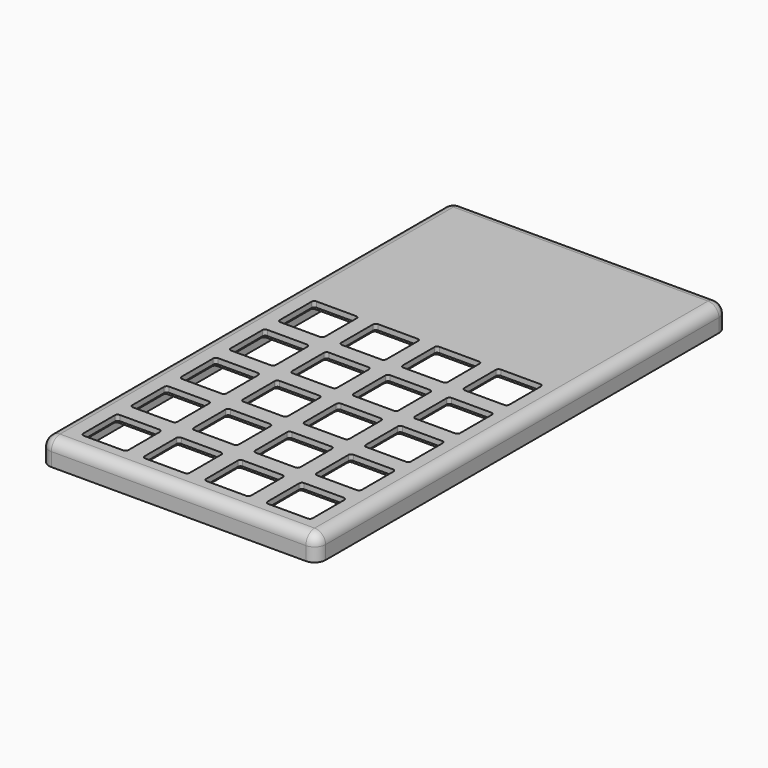
from build123d import *

# Parameters (mm, degrees)
F0_W         = 80.3275
F0_H         = 149.225
F1_DEPTH     = 7.14375
F2_R         = 3.175
F3_T1_DEPTH  = 11.90625
F3_S5_W      = 3.175
F3_S5_H      = 3.175
F3_T6_DEPTH  = 3.175
F3_S11_W     = 3.175
F3_S11_H     = 3.175
F3_T12_DEPTH = 3.175
F3_S17_W     = 3.175
F3_S17_H     = 3.175
F3_T18_DEPTH = 3.175
F3_S23_W     = 3.175
F3_S23_H     = 3.175
F3_T24_DEPTH = 3.175
F4_W         = 71.59625
F4_H         = 142.875
F5_DEPTH     = 5.55625
F7_DEPTH     = 25.4
F1_FACE_W    = 71.59625
F1_FACE_H    = 142.875
F9_DEPTH     = 25.4
F11_DEPTH    = 1.5875
F12_W        = 6.35
F12_H        = 1.984375
F12_W_2      = 12.7
F12_H_2      = 1.5875
F13_DEPTH    = 6.35


# Not quite as in the source:
# - a fillet or chamfer that OpenCascade refuses, or shapes differently, is made with other operations: its cross-section is extruded or revolved along the edge and cut away or added


with BuildPart() as f1:
    # F0 (on Top) → F1 (new body)
    with BuildSketch(Plane.XY):
        Rectangle(F0_W, F0_H)
    extrude(amount=F1_DEPTH)

    # F2
    f2_edges = [f1.edges().sort_by_distance(p)[0] for p in [
        (-40.16375, 0, 7.14375),
        (0, 74.6125, 7.14375),
        (40.16375, 0, 7.14375),
        (0, -74.6125, 7.14375),
    ]]
    fillet(f2_edges, radius=F2_R)

    # F3: fillet of radius 3.175 on 4 edges, made by hand

    # F3_s2 → F3_t1 (cut)
    with BuildSketch(Plane.XY.offset(-7.9375)):
        with BuildLine():
            ThreePointArc((40.16375, 71.4375), (39.2338140303, 73.6825640303), (36.98875, 74.6125))
            Line((36.98875, 74.6125), (40.16375, 74.6125))
            Line((40.16375, 74.6125), (40.16375, 71.4375))
        make_face()
        with BuildLine():
            ThreePointArc((40.16375, -71.4375), (39.2338140303, -73.6825640303), (36.98875, -74.6125))
            Line((36.98875, -74.6125), (40.16375, -74.6125))
            Line((40.16375, -74.6125), (40.16375, -71.4375))
        make_face()
        with BuildLine():
            ThreePointArc((-36.98875, -74.6125), (-39.2338140303, -73.6825640303), (-40.16375, -71.4375))
            Line((-40.16375, -71.4375), (-40.16375, -74.6125))
            Line((-40.16375, -74.6125), (-36.98875, -74.6125))
        make_face()
        with BuildLine():
            ThreePointArc((-36.98875, 74.6125), (-39.2338140303, 73.6825640303), (-40.16375, 71.4375))
            Line((-40.16375, 71.4375), (-40.16375, 74.6125))
            Line((-40.16375, 74.6125), (-36.98875, 74.6125))
        make_face()
    extrude(amount=F3_T1_DEPTH, mode=Mode.SUBTRACT)


with BuildPart() as f3_tool4:
    # F3_s5 → F3_t6 (new body)
    with BuildSketch(Plane.XZ.offset(-71.4375)):
        with Locations((-38.57625, 5.55625)):
            Rectangle(F3_S5_W, F3_S5_H)
    extrude(amount=-F3_T6_DEPTH)

    # F3_s7 → F3_t8 (revolve, cut)
    with BuildSketch(Plane(origin=(-36.98875, 71.4375, 3.96875), x_dir=(0.7071067812, 0, -0.7071067812), z_dir=(0.7071067812, 0, 0.7071067812))):
        with BuildLine():
            ThreePointArc((0, -3.175), (3.175, 0), (0, 3.175))
            Line((0, 3.175), (0, -3.175))
        make_face()
    revolve(axis=Axis((-36.98875, 71.4375, 3.96875), (0, 1, 0)), mode=Mode.SUBTRACT)


with BuildPart() as f1_1:
    add(f1.part)

    # F3_t3: cut F3_tool4
    add(f3_tool4.part, mode=Mode.SUBTRACT)


with BuildPart() as f3_tool10:
    # F3_s11 → F3_t12 (new body)
    with BuildSketch(Plane.XZ.offset(71.4375)):
        with Locations((-38.57625, 5.55625)):
            Rectangle(F3_S11_W, F3_S11_H)
    extrude(amount=F3_T12_DEPTH)

    # F3_s13 → F3_t14 (revolve, cut)
    with BuildSketch(Plane(origin=(-36.98875, -71.4375, 3.96875), x_dir=(0.7071067812, 0, -0.7071067812), z_dir=(-0.7071067812, 0, -0.7071067812))):
        with BuildLine():
            ThreePointArc((0, -3.175), (3.175, 0), (0, 3.175))
            Line((0, 3.175), (0, -3.175))
        make_face()
    revolve(axis=Axis((-36.98875, -71.4375, 3.96875), (0, -1, 0)), mode=Mode.SUBTRACT)


with BuildPart() as f1_2:
    add(f1_1.part)

    # F3_t9: cut F3_tool10
    add(f3_tool10.part, mode=Mode.SUBTRACT)


with BuildPart() as f3_tool16:
    # F3_s17 → F3_t18 (new body)
    with BuildSketch(Plane.YZ.offset(36.98875)):
        with Locations((-73.025, 5.55625)):
            Rectangle(F3_S17_W, F3_S17_H)
    extrude(amount=F3_T18_DEPTH)

    # F3_s19 → F3_t20 (revolve, cut)
    with BuildSketch(Plane(origin=(36.98875, -71.4375, 3.96875), x_dir=(0, 0.7071067812, -0.7071067812), z_dir=(0, -0.7071067812, -0.7071067812))):
        with BuildLine():
            ThreePointArc((0, -3.175), (3.175, 0), (0, 3.175))
            Line((0, 3.175), (0, -3.175))
        make_face()
    revolve(axis=Axis((36.98875, -71.4375, 3.96875), (1, 0, 0)), mode=Mode.SUBTRACT)


with BuildPart() as f1_3:
    add(f1_2.part)

    # F3_t15: cut F3_tool16
    add(f3_tool16.part, mode=Mode.SUBTRACT)


with BuildPart() as f3_tool22:
    # F3_s23 → F3_t24 (new body)
    with BuildSketch(Plane.YZ.offset(36.98875)):
        with Locations((73.025, 5.55625)):
            Rectangle(F3_S23_W, F3_S23_H)
    extrude(amount=F3_T24_DEPTH)

    # F3_s25 → F3_t26 (revolve, cut)
    with BuildSketch(Plane(origin=(36.98875, 71.4375, 3.96875), x_dir=(0, -0.7071067812, -0.7071067812), z_dir=(0, -0.7071067812, 0.7071067812))):
        with BuildLine():
            ThreePointArc((0, -3.175), (3.175, 0), (0, 3.175))
            Line((0, 3.175), (0, -3.175))
        make_face()
    revolve(axis=Axis((36.98875, 71.4375, 3.96875), (1, 0, 0)), mode=Mode.SUBTRACT)


with BuildPart() as f1_4:
    add(f1_3.part)

    # F3_t21: cut F3_tool22
    add(f3_tool22.part, mode=Mode.SUBTRACT)

    # F4 (on face) → F5 (cut)
    with BuildSketch(Plane(origin=(0, 0, 0), x_dir=(1, 0, 0), z_dir=(0, 0, -1))):
        with Locations((-1.190625, 0)):
            Rectangle(F4_W, F4_H)
    extrude(amount=-F5_DEPTH, mode=Mode.SUBTRACT)

    # F6 (on face) → F7 (cut)
    with BuildSketch(Plane.XY.offset(7.14375)):
        with BuildLine():
            Line((-33.0723875, 15.0256875), (-33.0723875, 3.5163125))
            ThreePointArc((-33.0723875, 3.5163125), (-32.8399035076, 2.9550464924), (-32.2786375, 2.7225625))
            Line((-32.2786375, 2.7225625), (-20.7692625, 2.7225625))
            ThreePointArc((-20.7692625, 2.7225625), (-20.2079964924, 2.9550464924), (-19.9755125, 3.5163125))
            Line((-19.9755125, 3.5163125), (-19.9755125, 15.0256875))
            ThreePointArc((-19.9755125, 15.0256875), (-20.2079964924, 15.5869535076), (-20.7692625, 15.8194375))
            Line((-20.7692625, 15.8194375), (-32.2786375, 15.8194375))
            ThreePointArc((-32.2786375, 15.8194375), (-32.8399035076, 15.5869535076), (-33.0723875, 15.0256875))
        make_face()
        with BuildLine():
            Line((-2.9130625, 15.8194375), (-14.4224375, 15.8194375))
            ThreePointArc((-14.4224375, 15.8194375), (-14.9837035076, 15.5869535076), (-15.2161875, 15.0256875))
            Line((-15.2161875, 15.0256875), (-15.2161875, 3.5163125))
            ThreePointArc((-15.2161875, 3.5163125), (-14.9837035076, 2.9550464924), (-14.4224375, 2.7225625))
            Line((-14.4224375, 2.7225625), (-2.9130625, 2.7225625))
            ThreePointArc((-2.9130625, 2.7225625), (-2.3517964924, 2.9550464924), (-2.1193125, 3.5163125))
            Line((-2.1193125, 3.5163125), (-2.1193125, 15.0256875))
            ThreePointArc((-2.1193125, 15.0256875), (-2.3517964924, 15.5869535076), (-2.9130625, 15.8194375))
        make_face()
        with BuildLine():
            Line((2.6400125, 15.0256875), (2.6400125, 3.5163125))
            ThreePointArc((2.6400125, 3.5163125), (2.8724964924, 2.9550464924), (3.4337625, 2.7225625))
            Line((3.4337625, 2.7225625), (14.9431375, 2.7225625))
            ThreePointArc((14.9431375, 2.7225625), (15.5044035076, 2.9550464924), (15.7368875, 3.5163125))
            Line((15.7368875, 3.5163125), (15.7368875, 15.0256875))
            ThreePointArc((15.7368875, 15.0256875), (15.5044035076, 15.5869535076), (14.9431375, 15.8194375))
            Line((14.9431375, 15.8194375), (3.4337625, 15.8194375))
            ThreePointArc((3.4337625, 15.8194375), (2.8724964924, 15.5869535076), (2.6400125, 15.0256875))
        make_face()
        with BuildLine():
            Line((20.4962125, 15.0256875), (20.4962125, 3.5163125))
            ThreePointArc((20.4962125, 3.5163125), (20.7286964924, 2.9550464924), (21.2899625, 2.7225625))
            Line((21.2899625, 2.7225625), (32.7993375, 2.7225625))
            ThreePointArc((32.7993375, 2.7225625), (33.3606035076, 2.9550464924), (33.5930875, 3.5163125))
            Line((33.5930875, 3.5163125), (33.5930875, 15.0256875))
            ThreePointArc((33.5930875, 15.0256875), (33.3606035076, 15.5869535076), (32.7993375, 15.8194375))
            Line((32.7993375, 15.8194375), (21.2899625, 15.8194375))
            ThreePointArc((21.2899625, 15.8194375), (20.7286964924, 15.5869535076), (20.4962125, 15.0256875))
        make_face()
        with BuildLine():
            Line((20.4962125, -2.8336875), (20.4962125, -14.3430625))
            ThreePointArc((20.4962125, -14.3430625), (20.7286964924, -14.9043285076), (21.2899625, -15.1368125))
            Line((21.2899625, -15.1368125), (32.7993375, -15.1368125))
            ThreePointArc((32.7993375, -15.1368125), (33.3606035076, -14.9043285076), (33.5930875, -14.3430625))
            Line((33.5930875, -14.3430625), (33.5930875, -2.8336875))
            ThreePointArc((33.5930875, -2.8336875), (33.3606035076, -2.2724214924), (32.7993375, -2.0399375))
            Line((32.7993375, -2.0399375), (21.2899625, -2.0399375))
            ThreePointArc((21.2899625, -2.0399375), (20.7286964924, -2.2724214924), (20.4962125, -2.8336875))
        make_face()
        with BuildLine():
            Line((2.6400125, -2.8336875), (2.6400125, -14.3430625))
            ThreePointArc((2.6400125, -14.3430625), (2.8724964924, -14.9043285076), (3.4337625, -15.1368125))
            Line((3.4337625, -15.1368125), (14.9431375, -15.1368125))
            ThreePointArc((14.9431375, -15.1368125), (15.5044035076, -14.9043285076), (15.7368875, -14.3430625))
            Line((15.7368875, -14.3430625), (15.7368875, -2.8336875))
            ThreePointArc((15.7368875, -2.8336875), (15.5044035076, -2.2724214924), (14.9431375, -2.0399375))
            Line((14.9431375, -2.0399375), (3.4337625, -2.0399375))
            ThreePointArc((3.4337625, -2.0399375), (2.8724964924, -2.2724214924), (2.6400125, -2.8336875))
        make_face()
        with BuildLine():
            Line((-2.9130625, -2.0399375), (-14.4224375, -2.0399375))
            ThreePointArc((-14.4224375, -2.0399375), (-14.9837035076, -2.2724214924), (-15.2161875, -2.8336875))
            Line((-15.2161875, -2.8336875), (-15.2161875, -14.3430625))
            ThreePointArc((-15.2161875, -14.3430625), (-14.9837035076, -14.9043285076), (-14.4224375, -15.1368125))
            Line((-14.4224375, -15.1368125), (-2.9130625, -15.1368125))
            ThreePointArc((-2.9130625, -15.1368125), (-2.3517964924, -14.9043285076), (-2.1193125, -14.3430625))
            Line((-2.1193125, -14.3430625), (-2.1193125, -2.8336875))
            ThreePointArc((-2.1193125, -2.8336875), (-2.3517964924, -2.2724214924), (-2.9130625, -2.0399375))
        make_face()
        with BuildLine():
            Line((-33.0723875, -2.8336875), (-33.0723875, -14.3430625))
            ThreePointArc((-33.0723875, -14.3430625), (-32.8399035076, -14.9043285076), (-32.2786375, -15.1368125))
            Line((-32.2786375, -15.1368125), (-20.7692625, -15.1368125))
            ThreePointArc((-20.7692625, -15.1368125), (-20.2079964924, -14.9043285076), (-19.9755125, -14.3430625))
            Line((-19.9755125, -14.3430625), (-19.9755125, -2.8336875))
            ThreePointArc((-19.9755125, -2.8336875), (-20.2079964924, -2.2724214924), (-20.7692625, -2.0399375))
            Line((-20.7692625, -2.0399375), (-32.2786375, -2.0399375))
            ThreePointArc((-32.2786375, -2.0399375), (-32.8399035076, -2.2724214924), (-33.0723875, -2.8336875))
        make_face()
        with BuildLine():
            Line((-33.0723875, -20.6930625), (-33.0723875, -32.2024375))
            ThreePointArc((-33.0723875, -32.2024375), (-32.8399035076, -32.7637035076), (-32.2786375, -32.9961875))
            Line((-32.2786375, -32.9961875), (-20.7692625, -32.9961875))
            ThreePointArc((-20.7692625, -32.9961875), (-20.2079964924, -32.7637035076), (-19.9755125, -32.2024375))
            Line((-19.9755125, -32.2024375), (-19.9755125, -20.6930625))
            ThreePointArc((-19.9755125, -20.6930625), (-20.2079964924, -20.1317964924), (-20.7692625, -19.8993125))
            Line((-20.7692625, -19.8993125), (-32.2786375, -19.8993125))
            ThreePointArc((-32.2786375, -19.8993125), (-32.8399035076, -20.1317964924), (-33.0723875, -20.6930625))
        make_face()
        with BuildLine():
            Line((-2.9130625, -19.8993125), (-14.4224375, -19.8993125))
            ThreePointArc((-14.4224375, -19.8993125), (-14.9837035076, -20.1317964924), (-15.2161875, -20.6930625))
            Line((-15.2161875, -20.6930625), (-15.2161875, -32.2024375))
            ThreePointArc((-15.2161875, -32.2024375), (-14.9837035076, -32.7637035076), (-14.4224375, -32.9961875))
            Line((-14.4224375, -32.9961875), (-2.9130625, -32.9961875))
            ThreePointArc((-2.9130625, -32.9961875), (-2.3517964924, -32.7637035076), (-2.1193125, -32.2024375))
            Line((-2.1193125, -32.2024375), (-2.1193125, -20.6930625))
            ThreePointArc((-2.1193125, -20.6930625), (-2.3517964924, -20.1317964924), (-2.9130625, -19.8993125))
        make_face()
        with BuildLine():
            Line((2.6400125, -20.6930625), (2.6400125, -32.2024375))
            ThreePointArc((2.6400125, -32.2024375), (2.8724964924, -32.7637035076), (3.4337625, -32.9961875))
            Line((3.4337625, -32.9961875), (14.9431375, -32.9961875))
            ThreePointArc((14.9431375, -32.9961875), (15.5044035076, -32.7637035076), (15.7368875, -32.2024375))
            Line((15.7368875, -32.2024375), (15.7368875, -20.6930625))
            ThreePointArc((15.7368875, -20.6930625), (15.5044035076, -20.1317964924), (14.9431375, -19.8993125))
            Line((14.9431375, -19.8993125), (3.4337625, -19.8993125))
            ThreePointArc((3.4337625, -19.8993125), (2.8724964924, -20.1317964924), (2.6400125, -20.6930625))
        make_face()
        with BuildLine():
            Line((20.4962125, -20.6930625), (20.4962125, -32.2024375))
            ThreePointArc((20.4962125, -32.2024375), (20.7286964924, -32.7637035076), (21.2899625, -32.9961875))
            Line((21.2899625, -32.9961875), (32.7993375, -32.9961875))
            ThreePointArc((32.7993375, -32.9961875), (33.3606035076, -32.7637035076), (33.5930875, -32.2024375))
            Line((33.5930875, -32.2024375), (33.5930875, -20.6930625))
            ThreePointArc((33.5930875, -20.6930625), (33.3606035076, -20.1317964924), (32.7993375, -19.8993125))
            Line((32.7993375, -19.8993125), (21.2899625, -19.8993125))
            ThreePointArc((21.2899625, -19.8993125), (20.7286964924, -20.1317964924), (20.4962125, -20.6930625))
        make_face()
        with BuildLine():
            Line((20.4962125, -38.5524375), (20.4962125, -50.0618125))
            ThreePointArc((20.4962125, -50.0618125), (20.7286964924, -50.6230785076), (21.2899625, -50.8555625))
            Line((21.2899625, -50.8555625), (32.7993375, -50.8555625))
            ThreePointArc((32.7993375, -50.8555625), (33.3606035076, -50.6230785076), (33.5930875, -50.0618125))
            Line((33.5930875, -50.0618125), (33.5930875, -38.5524375))
            ThreePointArc((33.5930875, -38.5524375), (33.3606035076, -37.9911714924), (32.7993375, -37.7586875))
            Line((32.7993375, -37.7586875), (21.2899625, -37.7586875))
            ThreePointArc((21.2899625, -37.7586875), (20.7286964924, -37.9911714924), (20.4962125, -38.5524375))
        make_face()
        with BuildLine():
            Line((2.6400125, -38.5524375), (2.6400125, -50.0618125))
            ThreePointArc((2.6400125, -50.0618125), (2.8724964924, -50.6230785076), (3.4337625, -50.8555625))
            Line((3.4337625, -50.8555625), (14.9431375, -50.8555625))
            ThreePointArc((14.9431375, -50.8555625), (15.5044035076, -50.6230785076), (15.7368875, -50.0618125))
            Line((15.7368875, -50.0618125), (15.7368875, -38.5524375))
            ThreePointArc((15.7368875, -38.5524375), (15.5044035076, -37.9911714924), (14.9431375, -37.7586875))
            Line((14.9431375, -37.7586875), (3.4337625, -37.7586875))
            ThreePointArc((3.4337625, -37.7586875), (2.8724964924, -37.9911714924), (2.6400125, -38.5524375))
        make_face()
        with BuildLine():
            Line((-2.9130625, -37.7586875), (-14.4224375, -37.7586875))
            ThreePointArc((-14.4224375, -37.7586875), (-14.9837035076, -37.9911714924), (-15.2161875, -38.5524375))
            Line((-15.2161875, -38.5524375), (-15.2161875, -50.0618125))
            ThreePointArc((-15.2161875, -50.0618125), (-14.9837035076, -50.6230785076), (-14.4224375, -50.8555625))
            Line((-14.4224375, -50.8555625), (-2.9130625, -50.8555625))
            ThreePointArc((-2.9130625, -50.8555625), (-2.3517964924, -50.6230785076), (-2.1193125, -50.0618125))
            Line((-2.1193125, -50.0618125), (-2.1193125, -38.5524375))
            ThreePointArc((-2.1193125, -38.5524375), (-2.3517964924, -37.9911714924), (-2.9130625, -37.7586875))
        make_face()
        with BuildLine():
            Line((-33.0723875, -38.5524375), (-33.0723875, -50.0618125))
            ThreePointArc((-33.0723875, -50.0618125), (-32.8399035076, -50.6230785076), (-32.2786375, -50.8555625))
            Line((-32.2786375, -50.8555625), (-20.7692625, -50.8555625))
            ThreePointArc((-20.7692625, -50.8555625), (-20.2079964924, -50.6230785076), (-19.9755125, -50.0618125))
            Line((-19.9755125, -50.0618125), (-19.9755125, -38.5524375))
            ThreePointArc((-19.9755125, -38.5524375), (-20.2079964924, -37.9911714924), (-20.7692625, -37.7586875))
            Line((-20.7692625, -37.7586875), (-32.2786375, -37.7586875))
            ThreePointArc((-32.2786375, -37.7586875), (-32.8399035076, -37.9911714924), (-33.0723875, -38.5524375))
        make_face()
        with BuildLine():
            Line((-26.52395, -55.6180625), (-26.52395, -68.7149375))
            Line((-26.52395, -68.7149375), (-20.7692625, -68.7149375))
            ThreePointArc((-20.7692625, -68.7149375), (-20.2079964924, -68.4824535076), (-19.9755125, -67.9211875))
            Line((-19.9755125, -67.9211875), (-19.9755125, -56.4118125))
            ThreePointArc((-19.9755125, -56.4118125), (-20.2079964924, -55.8505464924), (-20.7692625, -55.6180625))
            Line((-20.7692625, -55.6180625), (-26.52395, -55.6180625))
        make_face()
        with BuildLine():
            Line((-15.2161875, -56.4118125), (-15.2161875, -67.9211875))
            ThreePointArc((-15.2161875, -67.9211875), (-14.9837035076, -68.4824535076), (-14.4224375, -68.7149375))
            Line((-14.4224375, -68.7149375), (-2.9130625, -68.7149375))
            ThreePointArc((-2.9130625, -68.7149375), (-2.3517964924, -68.4824535076), (-2.1193125, -67.9211875))
            Line((-2.1193125, -67.9211875), (-2.1193125, -56.4118125))
            ThreePointArc((-2.1193125, -56.4118125), (-2.3517964924, -55.8505464924), (-2.9130625, -55.6180625))
            Line((-2.9130625, -55.6180625), (-14.4224375, -55.6180625))
            ThreePointArc((-14.4224375, -55.6180625), (-14.9837035076, -55.8505464924), (-15.2161875, -56.4118125))
        make_face()
        with BuildLine():
            Line((2.6400125, -56.4118125), (2.6400125, -67.9211875))
            ThreePointArc((2.6400125, -67.9211875), (2.8724964924, -68.4824535076), (3.4337625, -68.7149375))
            Line((3.4337625, -68.7149375), (14.9431375, -68.7149375))
            ThreePointArc((14.9431375, -68.7149375), (15.5044035076, -68.4824535076), (15.7368875, -67.9211875))
            Line((15.7368875, -67.9211875), (15.7368875, -56.4118125))
            ThreePointArc((15.7368875, -56.4118125), (15.5044035076, -55.8505464924), (14.9431375, -55.6180625))
            Line((14.9431375, -55.6180625), (3.4337625, -55.6180625))
            ThreePointArc((3.4337625, -55.6180625), (2.8724964924, -55.8505464924), (2.6400125, -56.4118125))
        make_face()
        with BuildLine():
            Line((20.4962125, -62.1665), (27.04465, -62.1665))
            Line((27.04465, -62.1665), (33.5930875, -62.1665))
            Line((33.5930875, -62.1665), (33.5930875, -56.4118125))
            ThreePointArc((33.5930875, -56.4118125), (33.3606035076, -55.8505464924), (32.7993375, -55.6180625))
            Line((32.7993375, -55.6180625), (21.2899625, -55.6180625))
            ThreePointArc((21.2899625, -55.6180625), (20.7286964924, -55.8505464924), (20.4962125, -56.4118125))
            Line((20.4962125, -56.4118125), (20.4962125, -62.1665))
        make_face()
        with BuildLine():
            Line((-33.0723875, -56.4118125), (-33.0723875, -67.9211875))
            ThreePointArc((-33.0723875, -67.9211875), (-32.8399035076, -68.4824535076), (-32.2786375, -68.7149375))
            Line((-32.2786375, -68.7149375), (-26.52395, -68.7149375))
            Line((-26.52395, -68.7149375), (-26.52395, -55.6180625))
            Line((-26.52395, -55.6180625), (-32.2786375, -55.6180625))
            ThreePointArc((-32.2786375, -55.6180625), (-32.8399035076, -55.8505464924), (-33.0723875, -56.4118125))
        make_face()
        with BuildLine():
            Line((21.2899625, -68.7149375), (27.04465, -68.7149375))
            Line((27.04465, -68.7149375), (27.04465, -62.1665))
            Line((27.04465, -62.1665), (20.4962125, -62.1665))
            Line((20.4962125, -62.1665), (20.4962125, -67.9211875))
            ThreePointArc((20.4962125, -67.9211875), (20.7286964924, -68.4824535076), (21.2899625, -68.7149375))
        make_face()
        with BuildLine():
            Line((27.04465, -62.1665), (27.04465, -68.7149375))
            Line((27.04465, -68.7149375), (32.7993375, -68.7149375))
            ThreePointArc((32.7993375, -68.7149375), (33.3606035076, -68.4824535076), (33.5930875, -67.9211875))
            Line((33.5930875, -67.9211875), (33.5930875, -62.1665))
            Line((33.5930875, -62.1665), (27.04465, -62.1665))
        make_face()
    extrude(amount=-F7_DEPTH, mode=Mode.SUBTRACT)

    # F8 (on face) + F1_face (on face) → F9 (cut)
    with BuildSketch(Plane(origin=(0, 0, 5.55625), x_dir=(1, 0, 0), z_dir=(0, 0, -1))):
        with BuildLine():
            Line((34.6075, 70.2711487276), (34.6075, 71.4375))
            Line((34.6075, 71.4375), (-36.98875, 71.4375))
            Line((-36.98875, 71.4375), (-36.98875, -71.4375))
            Line((-36.98875, -71.4375), (34.6075, -71.4375))
            Line((34.6075, -71.4375), (34.6075, -17.3756487276))
            ThreePointArc((34.6075, -17.3756487276), (34.4982723758, -17.3990763795), (34.3868375, -17.4069375))
            Line((34.3868375, -17.4069375), (19.7024625, -17.4069375))
            ThreePointArc((19.7024625, -17.4069375), (19.1411964924, -17.1744535076), (18.9087125, -16.6131875))
            Line((18.9087125, -16.6131875), (18.9087125, -1.9288125))
            ThreePointArc((18.9087125, -1.9288125), (19.1411964924, -1.3675464924), (19.7024625, -1.1350625))
            Line((19.7024625, -1.1350625), (34.3868375, -1.1350625))
            ThreePointArc((34.3868375, -1.1350625), (34.4982723758, -1.1429236205), (34.6075, -1.1663512724))
            Line((34.6075, -1.1663512724), (34.6075, 0.4837262724))
            ThreePointArc((34.6075, 0.4837262724), (34.4982723758, 0.4602986205), (34.3868375, 0.4524375))
            Line((34.3868375, 0.4524375), (19.7024625, 0.4524375))
            ThreePointArc((19.7024625, 0.4524375), (19.1411964924, 0.6849214924), (18.9087125, 1.2461875))
            Line((18.9087125, 1.2461875), (18.9087125, 15.9305625))
            ThreePointArc((18.9087125, 15.9305625), (19.1411964924, 16.4918285076), (19.7024625, 16.7243125))
            Line((19.7024625, 16.7243125), (34.3868375, 16.7243125))
            ThreePointArc((34.3868375, 16.7243125), (34.4982723758, 16.7164513795), (34.6075, 16.6930237276))
            Line((34.6075, 16.6930237276), (34.6075, 18.3431012724))
            ThreePointArc((34.6075, 18.3431012724), (34.4982723758, 18.3196736205), (34.3868375, 18.3118125))
            Line((34.3868375, 18.3118125), (19.7024625, 18.3118125))
            ThreePointArc((19.7024625, 18.3118125), (19.1411964924, 18.5442964924), (18.9087125, 19.1055625))
            Line((18.9087125, 19.1055625), (18.9087125, 33.7899375))
            ThreePointArc((18.9087125, 33.7899375), (19.1411964924, 34.3512035076), (19.7024625, 34.5836875))
            Line((19.7024625, 34.5836875), (34.3868375, 34.5836875))
            ThreePointArc((34.3868375, 34.5836875), (34.4982723758, 34.5758263795), (34.6075, 34.5523987276))
            Line((34.6075, 34.5523987276), (34.6075, 36.1711875))
            Line((34.6075, 36.1711875), (19.7024625, 36.1711875))
            ThreePointArc((19.7024625, 36.1711875), (19.1411964924, 36.4036714924), (18.9087125, 36.9649375))
            Line((18.9087125, 36.9649375), (18.9087125, 51.6493125))
            ThreePointArc((18.9087125, 51.6493125), (19.1411964924, 52.2105785076), (19.7024625, 52.4430625))
            Line((19.7024625, 52.4430625), (34.3868375, 52.4430625))
            ThreePointArc((34.3868375, 52.4430625), (34.4982723758, 52.4352013795), (34.6075, 52.4117737276))
            Line((34.6075, 52.4117737276), (34.6075, 54.0618512724))
            ThreePointArc((34.6075, 54.0618512724), (34.4982723758, 54.0384236205), (34.3868375, 54.0305625))
            Line((34.3868375, 54.0305625), (19.7024625, 54.0305625))
            ThreePointArc((19.7024625, 54.0305625), (19.1411964924, 54.2630464924), (18.9087125, 54.8243125))
            Line((18.9087125, 54.8243125), (18.9087125, 69.5086875))
            ThreePointArc((18.9087125, 69.5086875), (19.1411964924, 70.0699535076), (19.7024625, 70.3024375))
            Line((19.7024625, 70.3024375), (34.3868375, 70.3024375))
            ThreePointArc((34.3868375, 70.3024375), (34.4982723758, 70.2945763795), (34.6075, 70.2711487276))
        make_face()
        with BuildLine():
            ThreePointArc((-34.6598875, -1.9288125), (-34.4274035076, -1.3675464924), (-33.8661375, -1.1350625))
            Line((-33.8661375, -1.1350625), (-19.1817625, -1.1350625))
            ThreePointArc((-19.1817625, -1.1350625), (-18.6204964924, -1.3675464924), (-18.3880125, -1.9288125))
            Line((-18.3880125, -1.9288125), (-18.3880125, -16.6131875))
            ThreePointArc((-18.3880125, -16.6131875), (-18.6204964924, -17.1744535076), (-19.1817625, -17.4069375))
            Line((-19.1817625, -17.4069375), (-33.8661375, -17.4069375))
            ThreePointArc((-33.8661375, -17.4069375), (-34.4274035076, -17.1744535076), (-34.6598875, -16.6131875))
            Line((-34.6598875, -16.6131875), (-34.6598875, -1.9288125))
        make_face(mode=Mode.SUBTRACT)
        with BuildLine():
            ThreePointArc((-16.8036875, -1.9288125), (-16.5712035076, -1.3675464924), (-16.0099375, -1.1350625))
            Line((-16.0099375, -1.1350625), (-1.3255625, -1.1350625))
            ThreePointArc((-1.3255625, -1.1350625), (-0.7642964924, -1.3675464924), (-0.5318125, -1.9288125))
            Line((-0.5318125, -1.9288125), (-0.5318125, -16.6131875))
            ThreePointArc((-0.5318125, -16.6131875), (-0.7642964924, -17.1744535076), (-1.3255625, -17.4069375))
            Line((-1.3255625, -17.4069375), (-16.0099375, -17.4069375))
            ThreePointArc((-16.0099375, -17.4069375), (-16.5712035076, -17.1744535076), (-16.8036875, -16.6131875))
            Line((-16.8036875, -16.6131875), (-16.8036875, -1.9288125))
        make_face(mode=Mode.SUBTRACT)
        with BuildLine():
            Line((16.5306375, -17.4069375), (1.8462625, -17.4069375))
            ThreePointArc((1.8462625, -17.4069375), (1.2849964924, -17.1744535076), (1.0525125, -16.6131875))
            Line((1.0525125, -16.6131875), (1.0525125, -1.9288125))
            ThreePointArc((1.0525125, -1.9288125), (1.2849964924, -1.3675464924), (1.8462625, -1.1350625))
            Line((1.8462625, -1.1350625), (16.5306375, -1.1350625))
            ThreePointArc((16.5306375, -1.1350625), (17.0919035076, -1.3675464924), (17.3243875, -1.9288125))
            Line((17.3243875, -1.9288125), (17.3243875, -16.6131875))
            ThreePointArc((17.3243875, -16.6131875), (17.0919035076, -17.1744535076), (16.5306375, -17.4069375))
        make_face(mode=Mode.SUBTRACT)
        with BuildLine():
            ThreePointArc((-33.8661375, 0.4524375), (-34.4274035076, 0.6849214924), (-34.6598875, 1.2461875))
            Line((-34.6598875, 1.2461875), (-34.6598875, 15.9305625))
            ThreePointArc((-34.6598875, 15.9305625), (-34.4274035076, 16.4918285076), (-33.8661375, 16.7243125))
            Line((-33.8661375, 16.7243125), (-19.1817625, 16.7243125))
            ThreePointArc((-19.1817625, 16.7243125), (-18.6204964924, 16.4918285076), (-18.3880125, 15.9305625))
            Line((-18.3880125, 15.9305625), (-18.3880125, 1.2461875))
            ThreePointArc((-18.3880125, 1.2461875), (-18.6204964924, 0.6849214924), (-19.1817625, 0.4524375))
            Line((-19.1817625, 0.4524375), (-33.8661375, 0.4524375))
        make_face(mode=Mode.SUBTRACT)
        with BuildLine():
            Line((-19.1817625, 18.3118125), (-33.8661375, 18.3118125))
            ThreePointArc((-33.8661375, 18.3118125), (-34.4274035076, 18.5442964924), (-34.6598875, 19.1055625))
            Line((-34.6598875, 19.1055625), (-34.6598875, 33.7899375))
            ThreePointArc((-34.6598875, 33.7899375), (-34.4274035076, 34.3512035076), (-33.8661375, 34.5836875))
            Line((-33.8661375, 34.5836875), (-19.1817625, 34.5836875))
            ThreePointArc((-19.1817625, 34.5836875), (-18.6204964924, 34.3512035076), (-18.3880125, 33.7899375))
            Line((-18.3880125, 33.7899375), (-18.3880125, 19.1055625))
            ThreePointArc((-18.3880125, 19.1055625), (-18.6204964924, 18.5442964924), (-19.1817625, 18.3118125))
        make_face(mode=Mode.SUBTRACT)
        with BuildLine():
            Line((-0.5318125, 15.9305625), (-0.5318125, 1.2461875))
            ThreePointArc((-0.5318125, 1.2461875), (-0.7642964924, 0.6849214924), (-1.3255625, 0.4524375))
            Line((-1.3255625, 0.4524375), (-16.0099375, 0.4524375))
            ThreePointArc((-16.0099375, 0.4524375), (-16.5712035076, 0.6849214924), (-16.8036875, 1.2461875))
            Line((-16.8036875, 1.2461875), (-16.8036875, 15.9305625))
            ThreePointArc((-16.8036875, 15.9305625), (-16.5712035076, 16.4918285076), (-16.0099375, 16.7243125))
            Line((-16.0099375, 16.7243125), (-1.3255625, 16.7243125))
            ThreePointArc((-1.3255625, 16.7243125), (-0.7642964924, 16.4918285076), (-0.5318125, 15.9305625))
        make_face(mode=Mode.SUBTRACT)
        with BuildLine():
            ThreePointArc((-16.8036875, 33.7899375), (-16.5712035076, 34.3512035076), (-16.0099375, 34.5836875))
            Line((-16.0099375, 34.5836875), (-1.3255625, 34.5836875))
            ThreePointArc((-1.3255625, 34.5836875), (-0.7642964924, 34.3512035076), (-0.5318125, 33.7899375))
            Line((-0.5318125, 33.7899375), (-0.5318125, 19.1055625))
            ThreePointArc((-0.5318125, 19.1055625), (-0.7642964924, 18.5442964924), (-1.3255625, 18.3118125))
            Line((-1.3255625, 18.3118125), (-16.0099375, 18.3118125))
            ThreePointArc((-16.0099375, 18.3118125), (-16.5712035076, 18.5442964924), (-16.8036875, 19.1055625))
            Line((-16.8036875, 19.1055625), (-16.8036875, 33.7899375))
        make_face(mode=Mode.SUBTRACT)
        with BuildLine():
            ThreePointArc((-34.6598875, 51.6493125), (-34.4274035076, 52.2105785076), (-33.8661375, 52.4430625))
            Line((-33.8661375, 52.4430625), (-19.1817625, 52.4430625))
            ThreePointArc((-19.1817625, 52.4430625), (-18.6204964924, 52.2105785076), (-18.3880125, 51.6493125))
            Line((-18.3880125, 51.6493125), (-18.3880125, 36.9649375))
            ThreePointArc((-18.3880125, 36.9649375), (-18.6204964924, 36.4036714924), (-19.1817625, 36.1711875))
            Line((-19.1817625, 36.1711875), (-33.8661375, 36.1711875))
            ThreePointArc((-33.8661375, 36.1711875), (-34.4274035076, 36.4036714924), (-34.6598875, 36.9649375))
            Line((-34.6598875, 36.9649375), (-34.6598875, 51.6493125))
        make_face(mode=Mode.SUBTRACT)
        with BuildLine():
            Line((-33.8661375, 70.3024375), (-19.1817625, 70.3024375))
            ThreePointArc((-19.1817625, 70.3024375), (-18.6204964924, 70.0699535076), (-18.3880125, 69.5086875))
            Line((-18.3880125, 69.5086875), (-18.3880125, 54.8243125))
            ThreePointArc((-18.3880125, 54.8243125), (-18.6204964924, 54.2630464924), (-19.1817625, 54.0305625))
            Line((-19.1817625, 54.0305625), (-33.8661375, 54.0305625))
            ThreePointArc((-33.8661375, 54.0305625), (-34.4274035076, 54.2630464924), (-34.6598875, 54.8243125))
            Line((-34.6598875, 54.8243125), (-34.6598875, 69.5086875))
            ThreePointArc((-34.6598875, 69.5086875), (-34.4274035076, 70.0699535076), (-33.8661375, 70.3024375))
        make_face(mode=Mode.SUBTRACT)
        with BuildLine():
            ThreePointArc((-16.8036875, 51.6493125), (-16.5712035076, 52.2105785076), (-16.0099375, 52.4430625))
            Line((-16.0099375, 52.4430625), (-1.3255625, 52.4430625))
            ThreePointArc((-1.3255625, 52.4430625), (-0.7642964924, 52.2105785076), (-0.5318125, 51.6493125))
            Line((-0.5318125, 51.6493125), (-0.5318125, 36.9649375))
            ThreePointArc((-0.5318125, 36.9649375), (-0.7642964924, 36.4036714924), (-1.3255625, 36.1711875))
            Line((-1.3255625, 36.1711875), (-16.0099375, 36.1711875))
            ThreePointArc((-16.0099375, 36.1711875), (-16.5712035076, 36.4036714924), (-16.8036875, 36.9649375))
            Line((-16.8036875, 36.9649375), (-16.8036875, 51.6493125))
        make_face(mode=Mode.SUBTRACT)
        with BuildLine():
            Line((-16.0099375, 70.3024375), (-1.3255625, 70.3024375))
            ThreePointArc((-1.3255625, 70.3024375), (-0.7642964924, 70.0699535076), (-0.5318125, 69.5086875))
            Line((-0.5318125, 69.5086875), (-0.5318125, 54.8243125))
            ThreePointArc((-0.5318125, 54.8243125), (-0.7642964924, 54.2630464924), (-1.3255625, 54.0305625))
            Line((-1.3255625, 54.0305625), (-16.0099375, 54.0305625))
            ThreePointArc((-16.0099375, 54.0305625), (-16.5712035076, 54.2630464924), (-16.8036875, 54.8243125))
            Line((-16.8036875, 54.8243125), (-16.8036875, 69.5086875))
            ThreePointArc((-16.8036875, 69.5086875), (-16.5712035076, 70.0699535076), (-16.0099375, 70.3024375))
        make_face(mode=Mode.SUBTRACT)
        with BuildLine():
            Line((17.3243875, 15.9305625), (17.3243875, 1.2461875))
            ThreePointArc((17.3243875, 1.2461875), (17.0919035076, 0.6849214924), (16.5306375, 0.4524375))
            Line((16.5306375, 0.4524375), (1.8462625, 0.4524375))
            ThreePointArc((1.8462625, 0.4524375), (1.2849964924, 0.6849214924), (1.0525125, 1.2461875))
            Line((1.0525125, 1.2461875), (1.0525125, 15.9305625))
            ThreePointArc((1.0525125, 15.9305625), (1.2849964924, 16.4918285076), (1.8462625, 16.7243125))
            Line((1.8462625, 16.7243125), (16.5306375, 16.7243125))
            ThreePointArc((16.5306375, 16.7243125), (17.0919035076, 16.4918285076), (17.3243875, 15.9305625))
        make_face(mode=Mode.SUBTRACT)
        with BuildLine():
            ThreePointArc((1.0525125, 33.7899375), (1.2849964924, 34.3512035076), (1.8462625, 34.5836875))
            Line((1.8462625, 34.5836875), (16.5306375, 34.5836875))
            ThreePointArc((16.5306375, 34.5836875), (17.0919035076, 34.3512035076), (17.3243875, 33.7899375))
            Line((17.3243875, 33.7899375), (17.3243875, 19.1055625))
            ThreePointArc((17.3243875, 19.1055625), (17.0919035076, 18.5442964924), (16.5306375, 18.3118125))
            Line((16.5306375, 18.3118125), (1.8462625, 18.3118125))
            ThreePointArc((1.8462625, 18.3118125), (1.2849964924, 18.5442964924), (1.0525125, 19.1055625))
            Line((1.0525125, 19.1055625), (1.0525125, 33.7899375))
        make_face(mode=Mode.SUBTRACT)
        with BuildLine():
            ThreePointArc((1.0525125, 51.6493125), (1.2849964924, 52.2105785076), (1.8462625, 52.4430625))
            Line((1.8462625, 52.4430625), (16.5306375, 52.4430625))
            ThreePointArc((16.5306375, 52.4430625), (17.0919035076, 52.2105785076), (17.3243875, 51.6493125))
            Line((17.3243875, 51.6493125), (17.3243875, 36.9649375))
            ThreePointArc((17.3243875, 36.9649375), (17.0919035076, 36.4036714924), (16.5306375, 36.1711875))
            Line((16.5306375, 36.1711875), (1.8462625, 36.1711875))
            ThreePointArc((1.8462625, 36.1711875), (1.2849964924, 36.4036714924), (1.0525125, 36.9649375))
            Line((1.0525125, 36.9649375), (1.0525125, 51.6493125))
        make_face(mode=Mode.SUBTRACT)
        with BuildLine():
            ThreePointArc((1.0525125, 69.5086875), (1.2849964924, 70.0699535076), (1.8462625, 70.3024375))
            Line((1.8462625, 70.3024375), (16.5306375, 70.3024375))
            ThreePointArc((16.5306375, 70.3024375), (17.0919035076, 70.0699535076), (17.3243875, 69.5086875))
            Line((17.3243875, 69.5086875), (17.3243875, 54.8243125))
            ThreePointArc((17.3243875, 54.8243125), (17.0919035076, 54.2630464924), (16.5306375, 54.0305625))
            Line((16.5306375, 54.0305625), (1.8462625, 54.0305625))
            ThreePointArc((1.8462625, 54.0305625), (1.2849964924, 54.2630464924), (1.0525125, 54.8243125))
            Line((1.0525125, 54.8243125), (1.0525125, 69.5086875))
        make_face(mode=Mode.SUBTRACT)
        with BuildLine():
            ThreePointArc((35.1805875, 69.5086875), (35.0213412123, 69.9855984996), (34.6075, 70.2711487276))
            Line((34.6075, 70.2711487276), (34.6075, 54.0618512724))
            ThreePointArc((34.6075, 54.0618512724), (35.0213412123, 54.3474015004), (35.1805875, 54.8243125))
            Line((35.1805875, 54.8243125), (35.1805875, 69.5086875))
        make_face()
        with BuildLine():
            Line((34.6075, 54.0618512724), (34.6075, 70.2711487276))
            ThreePointArc((34.6075, 70.2711487276), (34.4982723758, 70.2945763795), (34.3868375, 70.3024375))
            Line((34.3868375, 70.3024375), (19.7024625, 70.3024375))
            ThreePointArc((19.7024625, 70.3024375), (19.1411964924, 70.0699535076), (18.9087125, 69.5086875))
            Line((18.9087125, 69.5086875), (18.9087125, 54.8243125))
            ThreePointArc((18.9087125, 54.8243125), (19.1411964924, 54.2630464924), (19.7024625, 54.0305625))
            Line((19.7024625, 54.0305625), (34.3868375, 54.0305625))
            ThreePointArc((34.3868375, 54.0305625), (34.4982723758, 54.0384236205), (34.6075, 54.0618512724))
        make_face()
        with BuildLine():
            ThreePointArc((35.1805875, 51.6493125), (35.0213412123, 52.1262234996), (34.6075, 52.4117737276))
            Line((34.6075, 52.4117737276), (34.6075, 36.1711875))
            Line((34.6075, 36.1711875), (35.1805875, 36.1711875))
            Line((35.1805875, 36.1711875), (35.1805875, 51.6493125))
        make_face()
        with BuildLine():
            Line((34.6075, 36.1711875), (34.6075, 52.4117737276))
            ThreePointArc((34.6075, 52.4117737276), (34.4982723758, 52.4352013795), (34.3868375, 52.4430625))
            Line((34.3868375, 52.4430625), (19.7024625, 52.4430625))
            ThreePointArc((19.7024625, 52.4430625), (19.1411964924, 52.2105785076), (18.9087125, 51.6493125))
            Line((18.9087125, 51.6493125), (18.9087125, 36.9649375))
            ThreePointArc((18.9087125, 36.9649375), (19.1411964924, 36.4036714924), (19.7024625, 36.1711875))
            Line((19.7024625, 36.1711875), (34.6075, 36.1711875))
        make_face()
        with BuildLine():
            ThreePointArc((34.3868375, -17.4069375), (34.4982723758, -17.3990763795), (34.6075, -17.3756487276))
            Line((34.6075, -17.3756487276), (34.6075, -1.1663512724))
            ThreePointArc((34.6075, -1.1663512724), (34.4982723758, -1.1429236205), (34.3868375, -1.1350625))
            Line((34.3868375, -1.1350625), (19.7024625, -1.1350625))
            ThreePointArc((19.7024625, -1.1350625), (19.1411964924, -1.3675464924), (18.9087125, -1.9288125))
            Line((18.9087125, -1.9288125), (18.9087125, -16.6131875))
            ThreePointArc((18.9087125, -16.6131875), (19.1411964924, -17.1744535076), (19.7024625, -17.4069375))
            Line((19.7024625, -17.4069375), (34.3868375, -17.4069375))
        make_face()
        with BuildLine():
            Line((34.6075, -1.1663512724), (34.6075, -17.3756487276))
            ThreePointArc((34.6075, -17.3756487276), (35.0213412123, -17.0900984996), (35.1805875, -16.6131875))
            Line((35.1805875, -16.6131875), (35.1805875, -1.9288125))
            ThreePointArc((35.1805875, -1.9288125), (35.0213412123, -1.4519015004), (34.6075, -1.1663512724))
        make_face()
        with BuildLine():
            ThreePointArc((35.1805875, 33.7899375), (35.0213412123, 34.2668484996), (34.6075, 34.5523987276))
            Line((34.6075, 34.5523987276), (34.6075, 18.3431012724))
            ThreePointArc((34.6075, 18.3431012724), (35.0213412123, 18.6286515004), (35.1805875, 19.1055625))
            Line((35.1805875, 19.1055625), (35.1805875, 33.7899375))
        make_face()
        with BuildLine():
            Line((34.6075, 18.3431012724), (34.6075, 34.5523987276))
            ThreePointArc((34.6075, 34.5523987276), (34.4982723758, 34.5758263795), (34.3868375, 34.5836875))
            Line((34.3868375, 34.5836875), (19.7024625, 34.5836875))
            ThreePointArc((19.7024625, 34.5836875), (19.1411964924, 34.3512035076), (18.9087125, 33.7899375))
            Line((18.9087125, 33.7899375), (18.9087125, 19.1055625))
            ThreePointArc((18.9087125, 19.1055625), (19.1411964924, 18.5442964924), (19.7024625, 18.3118125))
            Line((19.7024625, 18.3118125), (34.3868375, 18.3118125))
            ThreePointArc((34.3868375, 18.3118125), (34.4982723758, 18.3196736205), (34.6075, 18.3431012724))
        make_face()
        with BuildLine():
            ThreePointArc((34.3868375, 0.4524375), (34.4982723758, 0.4602986205), (34.6075, 0.4837262724))
            Line((34.6075, 0.4837262724), (34.6075, 16.6930237276))
            ThreePointArc((34.6075, 16.6930237276), (34.4982723758, 16.7164513795), (34.3868375, 16.7243125))
            Line((34.3868375, 16.7243125), (19.7024625, 16.7243125))
            ThreePointArc((19.7024625, 16.7243125), (19.1411964924, 16.4918285076), (18.9087125, 15.9305625))
            Line((18.9087125, 15.9305625), (18.9087125, 1.2461875))
            ThreePointArc((18.9087125, 1.2461875), (19.1411964924, 0.6849214924), (19.7024625, 0.4524375))
            Line((19.7024625, 0.4524375), (34.3868375, 0.4524375))
        make_face()
        with BuildLine():
            Line((34.6075, 16.6930237276), (34.6075, 0.4837262724))
            ThreePointArc((34.6075, 0.4837262724), (35.0213412123, 0.7692765004), (35.1805875, 1.2461875))
            Line((35.1805875, 1.2461875), (35.1805875, 15.9305625))
            ThreePointArc((35.1805875, 15.9305625), (35.0213412123, 16.4074734996), (34.6075, 16.6930237276))
        make_face()
    with BuildSketch(Plane(origin=(0, 0, 0), x_dir=(1, 0, 0), z_dir=(0, 0, -1))):
        with BuildLine():
            ThreePointArc((40.16375, 71.4375), (39.2338140303, 73.6825640303), (36.98875, 74.6125))
            Line((36.98875, 74.6125), (-36.98875, 74.6125))
            ThreePointArc((-36.98875, 74.6125), (-39.2338140303, 73.6825640303), (-40.16375, 71.4375))
            Line((-40.16375, 71.4375), (-40.16375, -71.4375))
            ThreePointArc((-40.16375, -71.4375), (-39.2338140303, -73.6825640303), (-36.98875, -74.6125))
            Line((-36.98875, -74.6125), (36.98875, -74.6125))
            ThreePointArc((36.98875, -74.6125), (39.2338140303, -73.6825640303), (40.16375, -71.4375))
            Line((40.16375, -71.4375), (40.16375, 71.4375))
        make_face()
        with Locations((-1.190625, 0)):
            Rectangle(F1_FACE_W, F1_FACE_H, mode=Mode.SUBTRACT)
    extrude(amount=F9_DEPTH, mode=Mode.SUBTRACT)

    # F10 (on face) → F11 (join)
    with BuildSketch(Plane(origin=(0, 0, 5.55625), x_dir=(1, 0, 0), z_dir=(0, 0, -1))):
        with BuildLine():
            Line((-36.98875, 71.4375), (-36.98875, -20.9631435573))
            Line((-36.98875, -20.9631435573), (34.6075, -20.9631435573))
            Line((34.6075, -20.9631435573), (34.6075, -17.3756487276))
            ThreePointArc((34.6075, -17.3756487276), (34.4982723758, -17.3990763795), (34.3868375, -17.4069375))
            Line((34.3868375, -17.4069375), (19.7024625, -17.4069375))
            ThreePointArc((19.7024625, -17.4069375), (19.1411964924, -17.1744535076), (18.9087125, -16.6131875))
            Line((18.9087125, -16.6131875), (18.9087125, -1.9288125))
            ThreePointArc((18.9087125, -1.9288125), (19.1411964924, -1.3675464924), (19.7024625, -1.1350625))
            Line((19.7024625, -1.1350625), (34.3868375, -1.1350625))
            ThreePointArc((34.3868375, -1.1350625), (34.4982723758, -1.1429236205), (34.6075, -1.1663512724))
            Line((34.6075, -1.1663512724), (34.6075, 0.4837262724))
            ThreePointArc((34.6075, 0.4837262724), (34.4982723758, 0.4602986205), (34.3868375, 0.4524375))
            Line((34.3868375, 0.4524375), (19.7024625, 0.4524375))
            ThreePointArc((19.7024625, 0.4524375), (19.1411964924, 0.6849214924), (18.9087125, 1.2461875))
            Line((18.9087125, 1.2461875), (18.9087125, 15.9305625))
            ThreePointArc((18.9087125, 15.9305625), (19.1411964924, 16.4918285076), (19.7024625, 16.7243125))
            Line((19.7024625, 16.7243125), (34.3868375, 16.7243125))
            ThreePointArc((34.3868375, 16.7243125), (34.4982723758, 16.7164513795), (34.6075, 16.6930237276))
            Line((34.6075, 16.6930237276), (34.6075, 18.3431012724))
            ThreePointArc((34.6075, 18.3431012724), (34.4982723758, 18.3196736205), (34.3868375, 18.3118125))
            Line((34.3868375, 18.3118125), (19.7024625, 18.3118125))
            ThreePointArc((19.7024625, 18.3118125), (19.1411964924, 18.5442964924), (18.9087125, 19.1055625))
            Line((18.9087125, 19.1055625), (18.9087125, 33.7899375))
            ThreePointArc((18.9087125, 33.7899375), (19.1411964924, 34.3512035076), (19.7024625, 34.5836875))
            Line((19.7024625, 34.5836875), (34.3868375, 34.5836875))
            ThreePointArc((34.3868375, 34.5836875), (34.4982723758, 34.5758263795), (34.6075, 34.5523987276))
            Line((34.6075, 34.5523987276), (34.6075, 36.1711875))
            Line((34.6075, 36.1711875), (19.7024625, 36.1711875))
            ThreePointArc((19.7024625, 36.1711875), (19.1411964924, 36.4036714924), (18.9087125, 36.9649375))
            Line((18.9087125, 36.9649375), (18.9087125, 51.6493125))
            ThreePointArc((18.9087125, 51.6493125), (19.1411964924, 52.2105785076), (19.7024625, 52.4430625))
            Line((19.7024625, 52.4430625), (34.3868375, 52.4430625))
            ThreePointArc((34.3868375, 52.4430625), (34.4982723758, 52.4352013795), (34.6075, 52.4117737276))
            Line((34.6075, 52.4117737276), (34.6075, 54.0618512724))
            ThreePointArc((34.6075, 54.0618512724), (34.4982723758, 54.0384236205), (34.3868375, 54.0305625))
            Line((34.3868375, 54.0305625), (19.7024625, 54.0305625))
            ThreePointArc((19.7024625, 54.0305625), (19.1411964924, 54.2630464924), (18.9087125, 54.8243125))
            Line((18.9087125, 54.8243125), (18.9087125, 69.5086875))
            ThreePointArc((18.9087125, 69.5086875), (19.1411964924, 70.0699535076), (19.7024625, 70.3024375))
            Line((19.7024625, 70.3024375), (34.3868375, 70.3024375))
            ThreePointArc((34.3868375, 70.3024375), (34.4982723758, 70.2945763795), (34.6075, 70.2711487276))
            Line((34.6075, 70.2711487276), (34.6075, 71.4375))
            Line((34.6075, 71.4375), (-36.98875, 71.4375))
        make_face()
        with BuildLine():
            Line((-33.8661375, -1.1350625), (-19.1817625, -1.1350625))
            ThreePointArc((-19.1817625, -1.1350625), (-18.6204964924, -1.3675464924), (-18.3880125, -1.9288125))
            Line((-18.3880125, -1.9288125), (-18.3880125, -16.6131875))
            ThreePointArc((-18.3880125, -16.6131875), (-18.6204964924, -17.1744535076), (-19.1817625, -17.4069375))
            Line((-19.1817625, -17.4069375), (-33.8661375, -17.4069375))
            ThreePointArc((-33.8661375, -17.4069375), (-34.4274035076, -17.1744535076), (-34.6598875, -16.6131875))
            Line((-34.6598875, -16.6131875), (-34.6598875, -1.9288125))
            ThreePointArc((-34.6598875, -1.9288125), (-34.4274035076, -1.3675464924), (-33.8661375, -1.1350625))
        make_face(mode=Mode.SUBTRACT)
        with BuildLine():
            Line((-16.0099375, -1.1350625), (-1.3255625, -1.1350625))
            ThreePointArc((-1.3255625, -1.1350625), (-0.7642964924, -1.3675464924), (-0.5318125, -1.9288125))
            Line((-0.5318125, -1.9288125), (-0.5318125, -16.6131875))
            ThreePointArc((-0.5318125, -16.6131875), (-0.7642964924, -17.1744535076), (-1.3255625, -17.4069375))
            Line((-1.3255625, -17.4069375), (-16.0099375, -17.4069375))
            ThreePointArc((-16.0099375, -17.4069375), (-16.5712035076, -17.1744535076), (-16.8036875, -16.6131875))
            Line((-16.8036875, -16.6131875), (-16.8036875, -1.9288125))
            ThreePointArc((-16.8036875, -1.9288125), (-16.5712035076, -1.3675464924), (-16.0099375, -1.1350625))
        make_face(mode=Mode.SUBTRACT)
        with BuildLine():
            ThreePointArc((1.8462625, -17.4069375), (1.2849964924, -17.1744535076), (1.0525125, -16.6131875))
            Line((1.0525125, -16.6131875), (1.0525125, -1.9288125))
            ThreePointArc((1.0525125, -1.9288125), (1.2849964924, -1.3675464924), (1.8462625, -1.1350625))
            Line((1.8462625, -1.1350625), (16.5306375, -1.1350625))
            ThreePointArc((16.5306375, -1.1350625), (17.0919035076, -1.3675464924), (17.3243875, -1.9288125))
            Line((17.3243875, -1.9288125), (17.3243875, -16.6131875))
            ThreePointArc((17.3243875, -16.6131875), (17.0919035076, -17.1744535076), (16.5306375, -17.4069375))
            Line((16.5306375, -17.4069375), (1.8462625, -17.4069375))
        make_face(mode=Mode.SUBTRACT)
        with BuildLine():
            Line((-34.6598875, 1.2461875), (-34.6598875, 15.9305625))
            ThreePointArc((-34.6598875, 15.9305625), (-34.4274035076, 16.4918285076), (-33.8661375, 16.7243125))
            Line((-33.8661375, 16.7243125), (-19.1817625, 16.7243125))
            ThreePointArc((-19.1817625, 16.7243125), (-18.6204964924, 16.4918285076), (-18.3880125, 15.9305625))
            Line((-18.3880125, 15.9305625), (-18.3880125, 1.2461875))
            ThreePointArc((-18.3880125, 1.2461875), (-18.6204964924, 0.6849214924), (-19.1817625, 0.4524375))
            Line((-19.1817625, 0.4524375), (-33.8661375, 0.4524375))
            ThreePointArc((-33.8661375, 0.4524375), (-34.4274035076, 0.6849214924), (-34.6598875, 1.2461875))
        make_face(mode=Mode.SUBTRACT)
        with BuildLine():
            ThreePointArc((-33.8661375, 18.3118125), (-34.4274035076, 18.5442964924), (-34.6598875, 19.1055625))
            Line((-34.6598875, 19.1055625), (-34.6598875, 33.7899375))
            ThreePointArc((-34.6598875, 33.7899375), (-34.4274035076, 34.3512035076), (-33.8661375, 34.5836875))
            Line((-33.8661375, 34.5836875), (-19.1817625, 34.5836875))
            ThreePointArc((-19.1817625, 34.5836875), (-18.6204964924, 34.3512035076), (-18.3880125, 33.7899375))
            Line((-18.3880125, 33.7899375), (-18.3880125, 19.1055625))
            ThreePointArc((-18.3880125, 19.1055625), (-18.6204964924, 18.5442964924), (-19.1817625, 18.3118125))
            Line((-19.1817625, 18.3118125), (-33.8661375, 18.3118125))
        make_face(mode=Mode.SUBTRACT)
        with BuildLine():
            ThreePointArc((-0.5318125, 1.2461875), (-0.7642964924, 0.6849214924), (-1.3255625, 0.4524375))
            Line((-1.3255625, 0.4524375), (-16.0099375, 0.4524375))
            ThreePointArc((-16.0099375, 0.4524375), (-16.5712035076, 0.6849214924), (-16.8036875, 1.2461875))
            Line((-16.8036875, 1.2461875), (-16.8036875, 15.9305625))
            ThreePointArc((-16.8036875, 15.9305625), (-16.5712035076, 16.4918285076), (-16.0099375, 16.7243125))
            Line((-16.0099375, 16.7243125), (-1.3255625, 16.7243125))
            ThreePointArc((-1.3255625, 16.7243125), (-0.7642964924, 16.4918285076), (-0.5318125, 15.9305625))
            Line((-0.5318125, 15.9305625), (-0.5318125, 1.2461875))
        make_face(mode=Mode.SUBTRACT)
        with BuildLine():
            Line((-16.0099375, 34.5836875), (-1.3255625, 34.5836875))
            ThreePointArc((-1.3255625, 34.5836875), (-0.7642964924, 34.3512035076), (-0.5318125, 33.7899375))
            Line((-0.5318125, 33.7899375), (-0.5318125, 19.1055625))
            ThreePointArc((-0.5318125, 19.1055625), (-0.7642964924, 18.5442964924), (-1.3255625, 18.3118125))
            Line((-1.3255625, 18.3118125), (-16.0099375, 18.3118125))
            ThreePointArc((-16.0099375, 18.3118125), (-16.5712035076, 18.5442964924), (-16.8036875, 19.1055625))
            Line((-16.8036875, 19.1055625), (-16.8036875, 33.7899375))
            ThreePointArc((-16.8036875, 33.7899375), (-16.5712035076, 34.3512035076), (-16.0099375, 34.5836875))
        make_face(mode=Mode.SUBTRACT)
        with BuildLine():
            Line((-33.8661375, 52.4430625), (-19.1817625, 52.4430625))
            ThreePointArc((-19.1817625, 52.4430625), (-18.6204964924, 52.2105785076), (-18.3880125, 51.6493125))
            Line((-18.3880125, 51.6493125), (-18.3880125, 36.9649375))
            ThreePointArc((-18.3880125, 36.9649375), (-18.6204964924, 36.4036714924), (-19.1817625, 36.1711875))
            Line((-19.1817625, 36.1711875), (-33.8661375, 36.1711875))
            ThreePointArc((-33.8661375, 36.1711875), (-34.4274035076, 36.4036714924), (-34.6598875, 36.9649375))
            Line((-34.6598875, 36.9649375), (-34.6598875, 51.6493125))
            ThreePointArc((-34.6598875, 51.6493125), (-34.4274035076, 52.2105785076), (-33.8661375, 52.4430625))
        make_face(mode=Mode.SUBTRACT)
        with BuildLine():
            ThreePointArc((-19.1817625, 70.3024375), (-18.6204964924, 70.0699535076), (-18.3880125, 69.5086875))
            Line((-18.3880125, 69.5086875), (-18.3880125, 54.8243125))
            ThreePointArc((-18.3880125, 54.8243125), (-18.6204964924, 54.2630464924), (-19.1817625, 54.0305625))
            Line((-19.1817625, 54.0305625), (-33.8661375, 54.0305625))
            ThreePointArc((-33.8661375, 54.0305625), (-34.4274035076, 54.2630464924), (-34.6598875, 54.8243125))
            Line((-34.6598875, 54.8243125), (-34.6598875, 69.5086875))
            ThreePointArc((-34.6598875, 69.5086875), (-34.4274035076, 70.0699535076), (-33.8661375, 70.3024375))
            Line((-33.8661375, 70.3024375), (-19.1817625, 70.3024375))
        make_face(mode=Mode.SUBTRACT)
        with BuildLine():
            Line((-16.0099375, 52.4430625), (-1.3255625, 52.4430625))
            ThreePointArc((-1.3255625, 52.4430625), (-0.7642964924, 52.2105785076), (-0.5318125, 51.6493125))
            Line((-0.5318125, 51.6493125), (-0.5318125, 36.9649375))
            ThreePointArc((-0.5318125, 36.9649375), (-0.7642964924, 36.4036714924), (-1.3255625, 36.1711875))
            Line((-1.3255625, 36.1711875), (-16.0099375, 36.1711875))
            ThreePointArc((-16.0099375, 36.1711875), (-16.5712035076, 36.4036714924), (-16.8036875, 36.9649375))
            Line((-16.8036875, 36.9649375), (-16.8036875, 51.6493125))
            ThreePointArc((-16.8036875, 51.6493125), (-16.5712035076, 52.2105785076), (-16.0099375, 52.4430625))
        make_face(mode=Mode.SUBTRACT)
        with BuildLine():
            ThreePointArc((-1.3255625, 70.3024375), (-0.7642964924, 70.0699535076), (-0.5318125, 69.5086875))
            Line((-0.5318125, 69.5086875), (-0.5318125, 54.8243125))
            ThreePointArc((-0.5318125, 54.8243125), (-0.7642964924, 54.2630464924), (-1.3255625, 54.0305625))
            Line((-1.3255625, 54.0305625), (-16.0099375, 54.0305625))
            ThreePointArc((-16.0099375, 54.0305625), (-16.5712035076, 54.2630464924), (-16.8036875, 54.8243125))
            Line((-16.8036875, 54.8243125), (-16.8036875, 69.5086875))
            ThreePointArc((-16.8036875, 69.5086875), (-16.5712035076, 70.0699535076), (-16.0099375, 70.3024375))
            Line((-16.0099375, 70.3024375), (-1.3255625, 70.3024375))
        make_face(mode=Mode.SUBTRACT)
        with BuildLine():
            ThreePointArc((17.3243875, 1.2461875), (17.0919035076, 0.6849214924), (16.5306375, 0.4524375))
            Line((16.5306375, 0.4524375), (1.8462625, 0.4524375))
            ThreePointArc((1.8462625, 0.4524375), (1.2849964924, 0.6849214924), (1.0525125, 1.2461875))
            Line((1.0525125, 1.2461875), (1.0525125, 15.9305625))
            ThreePointArc((1.0525125, 15.9305625), (1.2849964924, 16.4918285076), (1.8462625, 16.7243125))
            Line((1.8462625, 16.7243125), (16.5306375, 16.7243125))
            ThreePointArc((16.5306375, 16.7243125), (17.0919035076, 16.4918285076), (17.3243875, 15.9305625))
            Line((17.3243875, 15.9305625), (17.3243875, 1.2461875))
        make_face(mode=Mode.SUBTRACT)
        with BuildLine():
            Line((1.8462625, 34.5836875), (16.5306375, 34.5836875))
            ThreePointArc((16.5306375, 34.5836875), (17.0919035076, 34.3512035076), (17.3243875, 33.7899375))
            Line((17.3243875, 33.7899375), (17.3243875, 19.1055625))
            ThreePointArc((17.3243875, 19.1055625), (17.0919035076, 18.5442964924), (16.5306375, 18.3118125))
            Line((16.5306375, 18.3118125), (1.8462625, 18.3118125))
            ThreePointArc((1.8462625, 18.3118125), (1.2849964924, 18.5442964924), (1.0525125, 19.1055625))
            Line((1.0525125, 19.1055625), (1.0525125, 33.7899375))
            ThreePointArc((1.0525125, 33.7899375), (1.2849964924, 34.3512035076), (1.8462625, 34.5836875))
        make_face(mode=Mode.SUBTRACT)
        with BuildLine():
            Line((1.8462625, 52.4430625), (16.5306375, 52.4430625))
            ThreePointArc((16.5306375, 52.4430625), (17.0919035076, 52.2105785076), (17.3243875, 51.6493125))
            Line((17.3243875, 51.6493125), (17.3243875, 36.9649375))
            ThreePointArc((17.3243875, 36.9649375), (17.0919035076, 36.4036714924), (16.5306375, 36.1711875))
            Line((16.5306375, 36.1711875), (1.8462625, 36.1711875))
            ThreePointArc((1.8462625, 36.1711875), (1.2849964924, 36.4036714924), (1.0525125, 36.9649375))
            Line((1.0525125, 36.9649375), (1.0525125, 51.6493125))
            ThreePointArc((1.0525125, 51.6493125), (1.2849964924, 52.2105785076), (1.8462625, 52.4430625))
        make_face(mode=Mode.SUBTRACT)
        with BuildLine():
            Line((1.8462625, 70.3024375), (16.5306375, 70.3024375))
            ThreePointArc((16.5306375, 70.3024375), (17.0919035076, 70.0699535076), (17.3243875, 69.5086875))
            Line((17.3243875, 69.5086875), (17.3243875, 54.8243125))
            ThreePointArc((17.3243875, 54.8243125), (17.0919035076, 54.2630464924), (16.5306375, 54.0305625))
            Line((16.5306375, 54.0305625), (1.8462625, 54.0305625))
            ThreePointArc((1.8462625, 54.0305625), (1.2849964924, 54.2630464924), (1.0525125, 54.8243125))
            Line((1.0525125, 54.8243125), (1.0525125, 69.5086875))
            ThreePointArc((1.0525125, 69.5086875), (1.2849964924, 70.0699535076), (1.8462625, 70.3024375))
        make_face(mode=Mode.SUBTRACT)
    extrude(amount=F11_DEPTH)

    # F12 (on face) → F13 (cut)
    with BuildSketch(Plane(origin=(-40.16375, 0, 0), x_dir=(0, -1, 0), z_dir=(-1, 0, 0))):
        Polygon((-38.97122, 0), (-38.97122, 3.96875), (-51.67122, 3.96875), (-51.67122, 1.984375), (-45.32122, 1.984375), (-45.32122, 0), align=None)
        with Locations((-48.49622, 0.9921875)):
            Rectangle(F12_W, F12_H)
        with Locations((-45.32122, 4.7625)):
            Rectangle(F12_W_2, F12_H_2)
    extrude(amount=-F13_DEPTH, mode=Mode.SUBTRACT)


solid = f1_4.part
